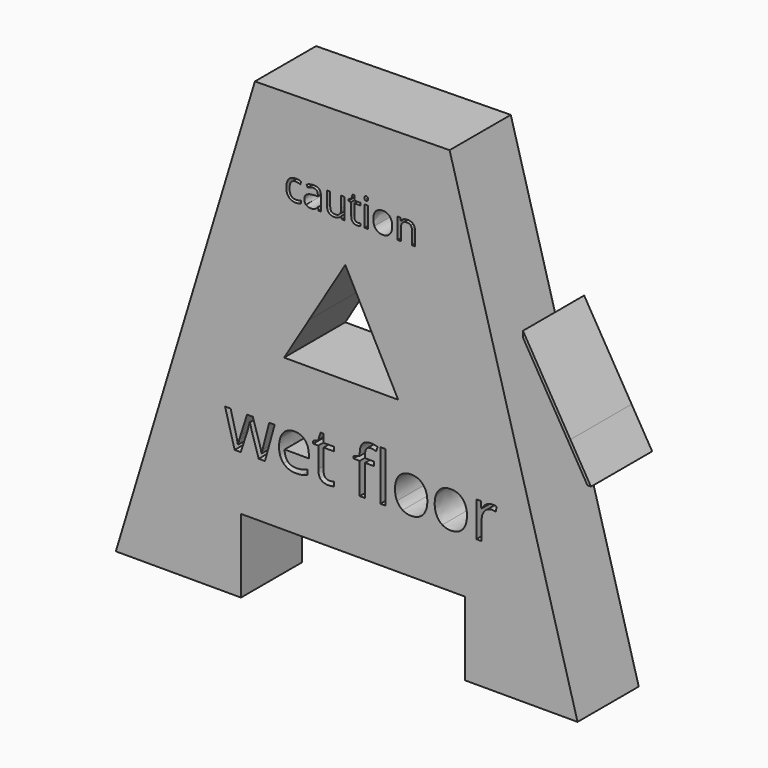
from build123d import *

# Parameters (mm, degrees)
F1_DEPTH = 12.7
F2_W     = 0.884249532
F2_H     = 8.2853670025
F2_W_2   = 0.5201468884
F2_H_2   = 3.4325685798
F3_DEPTH = 12.7


# Not quite as in the source:
# - a feature names something its author has since deleted; it is built from what else it names


with BuildPart() as f1:
    # F0 (on Front) → F1 (new body)
    with BuildSketch(Plane.XZ):
        with BuildLine():
            Line((9.6578345108, 21.5954678464), (6.4095085072, 27.0940973965))
            Line((6.4095085072, 27.0940973965), (6.4095085072, 26.0954775043))
            Line((6.4095085072, 26.0954775043), (9.3747755358, 21.0759982743))
            add(Edge.make_bspline(
                [(9.6578345108, 21.5954678464), (9.5118502558, 21.3402983679), (9.3747755358, 21.0759982743)],
                knots=[0.2874772556, 0.2874772556, 0.2874772556, 0.3442899073, 0.3442899073, 0.3442899073], degree=2))
        make_face()
        with BuildLine():
            Line((14.2873522737, 13.7588150149), (9.6578345108, 21.5954678464))
            add(Edge.make_bspline(
                [(9.6578345108, 21.5954678464), (9.5118502558, 21.3402983679), (9.3747755358, 21.0759982743)],
                knots=[0.2874772556, 0.2874772556, 0.2874772556, 0.3442899073, 0.3442899073, 0.3442899073], degree=2))
            Line((9.3747755358, 21.0759982743), (13.6974156478, 13.7588150149))
            Line((13.6974156478, 13.7588150149), (14.2873522737, 13.7588150149))
        make_face()
        Polygon((17.7024840034, 7.9778237518), (14.2873522737, 13.7588150149), (13.6974156478, 13.7588150149), (17.1125473775, 7.9778237518), align=None)
    extrude(amount=F1_DEPTH)


with BuildPart() as f3:
    # F2 (on Front) → F3 (new body)
    with BuildSketch(Plane.XZ):
        Polygon((-5.7727261446, 49.5300032198), (-38.1000004709, 49.0681789815), (-61.1909106374, -27.1318182349), (-40.4090918601, -27.1318182349), (-40.4090918601, -14.8936361074), (-3.2327286899, -14.8936361074), (-3.2327286899, -27.1318182349), (15.4709070921, -27.1318182349), align=None)
        Polygon((-47.3363660276, -7.9663638026), (-38.1000004709, 43.2954542339), (-7.398655434, 43.7340506074), (4.8490930349, -7.9663638026), align=None, mode=Mode.SUBTRACT)
        Polygon((-7.398655434, 43.7340506074), (-38.1000004709, 43.2954542339), (-47.3363660276, -7.9663638026), (4.8490930349, -7.9663638026), align=None)
        with BuildLine():
            Line((-36.4280137258, -5.8881817386), (-37.4775276213, -5.8881817386))
            Line((-37.4775276213, -5.8881817386), (-38.5474865926, -2.4653352841))
            add(Edge.make_bspline(
                [(-38.5474865926, -2.4653352841), (-38.649711972, -2.1501403642), (-38.9257204965, -1.0375874848)],
                knots=[0, 0, 0, 1, 1, 1], degree=2))
            Line((-38.9257204965, -1.0375874848), (-38.9683144046, -1.0375874848))
            add(Edge.make_bspline(
                [(-38.9683144046, -1.0375874848), (-39.1812839451, -1.9695421939), (-39.3414370395, -2.475557822)],
                knots=[0, 0, 0, 1, 1, 1], degree=2))
            Line((-39.3414370395, -2.475557822), (-40.443767381, -5.8881817386))
            Line((-40.443767381, -5.8881817386), (-41.4660211752, -5.8881817386))
            Line((-41.4660211752, -5.8881817386), (-43.0573295816, -0.0528163296))
            Line((-43.0573295816, -0.0528163296), (-42.1304861415, -0.0528163296))
            add(Edge.make_bspline(
                [(-42.1304861415, -0.0528163296), (-41.5665427983, -2.2523657436), (-41.2709410762, -3.4024012622)],
                knots=[0, 0, 0, 1, 1, 1], degree=2))
            add(Edge.make_bspline(
                [(-41.2709410762, -3.4024012622), (-40.975339354, -4.5524367807), (-40.9327454459, -4.9511157605)],
                knots=[0, 0, 0, 1, 1, 1], degree=2))
            Line((-40.9327454459, -4.9511157605), (-40.8901515378, -4.9511157605))
            add(Edge.make_bspline(
                [(-40.8901515378, -4.9511157605), (-40.8322238228, -4.6478471348), (-40.701886464, -4.1656840952)],
                knots=[0, 0, 0, 1, 1, 1], degree=2))
            add(Edge.make_bspline(
                [(-40.701886464, -4.1656840952), (-40.5715491053, -3.6835210556), (-40.4744349948, -3.4024012622)],
                knots=[0, 0, 0, 1, 1, 1], degree=2))
            Line((-40.4744349948, -3.4024012622), (-39.4044760235, -0.0528163296))
            Line((-39.4044760235, -0.0528163296), (-38.4469649695, -0.0528163296))
            Line((-38.4469649695, -0.0528163296), (-37.402562343, -3.4024012622))
            add(Edge.make_bspline(
                [(-37.402562343, -3.4024012622), (-37.1044049864, -4.317318408), (-36.9987720943, -4.9408932225)],
                knots=[0, 0, 0, 1, 1, 1], degree=2))
            Line((-36.9987720943, -4.9408932225), (-36.9561781862, -4.9408932225))
            add(Edge.make_bspline(
                [(-36.9561781862, -4.9408932225), (-36.934029354, -4.7483687579), (-36.8411746343, -4.3488379)],
                knots=[0, 0, 0, 1, 1, 1], degree=2))
            add(Edge.make_bspline(
                [(-36.8411746343, -4.3488379), (-36.7483199147, -3.9493070421), (-35.7311773894, -0.0528163296)],
                knots=[0, 0, 0, 1, 1, 1], degree=2))
            Line((-35.7311773894, -0.0528163296), (-34.8162602435, -0.0528163296))
            Line((-34.8162602435, -0.0528163296), (-36.4280137258, -5.8881817386))
        make_face(mode=Mode.SUBTRACT)
        with BuildLine():
            add(Edge.make_bspline(
                [(-30.2876759349, -5.9069230581), (-30.7050962343, -5.995518387), (-31.2962996786, -5.995518387)],
                knots=[0, 0, 0, 1, 1, 1], degree=2))
            add(Edge.make_bspline(
                [(-31.2962996786, -5.995518387), (-32.5894507284, -5.995518387), (-33.3382516327, -5.206679209)],
                knots=[0, 0, 0, 1, 1, 1], degree=2))
            add(Edge.make_bspline(
                [(-33.3382516327, -5.206679209), (-34.087052537, -4.4178400311), (-34.087052537, -3.0190560893)],
                knots=[0, 0, 0, 1, 1, 1], degree=2))
            add(Edge.make_bspline(
                [(-34.087052537, -3.0190560893), (-34.087052537, -1.6066420969), (-33.3919199569, -0.7760608891)],
                knots=[0, 0, 0, 1, 1, 1], degree=2))
            add(Edge.make_bspline(
                [(-33.3919199569, -0.7760608891), (-32.6967873768, 0.0545203188), (-31.524603026, 0.0545203188)],
                knots=[0, 0, 0, 1, 1, 1], degree=2))
            add(Edge.make_bspline(
                [(-31.524603026, 0.0545203188), (-30.4290877098, 0.0545203188), (-29.7901790884, -0.6670204843)],
                knots=[0, 0, 0, 1, 1, 1], degree=2))
            add(Edge.make_bspline(
                [(-29.7901790884, -0.6670204843), (-29.151270467, -1.3885612875), (-29.151270467, -2.5709681762)],
                knots=[0, 0, 0, 1, 1, 1], degree=2))
            Line((-29.151270467, -2.5709681762), (-29.151270467, -3.1298002504))
            Line((-29.151270467, -3.1298002504), (-33.1704316348, -3.1298002504))
            add(Edge.make_bspline(
                [(-33.1704316348, -3.1298002504), (-33.1431715336, -4.1571653136), (-32.650785956, -4.6895891648)],
                knots=[0, 0, 0, 1, 1, 1], degree=2))
            add(Edge.make_bspline(
                [(-32.650785956, -4.6895891648), (-32.1584003784, -5.222013016), (-31.2639283085, -5.222013016)],
                knots=[0, 0, 0, 1, 1, 1], degree=2))
            add(Edge.make_bspline(
                [(-31.2639283085, -5.222013016), (-30.3217510614, -5.222013016), (-29.4017226466, -4.8284453052)],
                knots=[0, 0, 0, 1, 1, 1], degree=2))
            Line((-29.4017226466, -4.8284453052), (-29.4017226466, -5.6172844831))
            add(Edge.make_bspline(
                [(-29.4017226466, -5.6172844831), (-29.8702556356, -5.8183277293), (-30.2876759349, -5.9069230581)],
                knots=[0, 0, 0, 1, 1, 1], degree=2))
        make_face(mode=Mode.SUBTRACT)
        with BuildLine():
            add(Edge.make_bspline(
                [(-26.4457054248, -4.9826352525), (-26.1952532452, -5.2646069241), (-25.7590916263, -5.2646069241)],
                knots=[0, 0, 0, 1, 1, 1], degree=2))
            add(Edge.make_bspline(
                [(-25.7590916263, -5.2646069241), (-25.5239732537, -5.2646069241), (-25.3058924442, -5.2305317976)],
                knots=[0, 0, 0, 1, 1, 1], degree=2))
            add(Edge.make_bspline(
                [(-25.3058924442, -5.2305317976), (-25.0878116348, -5.1964566711), (-24.9600299105, -5.158974032)],
                knots=[0, 0, 0, 1, 1, 1], degree=2))
            Line((-24.9600299105, -5.158974032), (-24.9600299105, -5.8353652925))
            add(Edge.make_bspline(
                [(-24.9600299105, -5.8353652925), (-25.1031454417, -5.9035155455), (-25.3825614788, -5.9495169662)],
                knots=[0, 0, 0, 1, 1, 1], degree=2))
            add(Edge.make_bspline(
                [(-25.3825614788, -5.9495169662), (-25.6619775159, -5.995518387), (-25.8868733506, -5.995518387)],
                knots=[0, 0, 0, 1, 1, 1], degree=2))
            add(Edge.make_bspline(
                [(-25.8868733506, -5.995518387), (-27.5787033801, -5.995518387), (-27.5787033801, -4.211685516)],
                knots=[0, 0, 0, 1, 1, 1], degree=2))
            Line((-27.5787033801, -4.211685516), (-27.5787033801, -0.7394301281))
            Line((-27.5787033801, -0.7394301281), (-28.4152477351, -0.7394301281))
            Line((-28.4152477351, -0.7394301281), (-28.4152477351, -0.3134910472))
            Line((-28.4152477351, -0.3134910472), (-27.5787033801, 0.0545203188))
            Line((-27.5787033801, 0.0545203188), (-27.2072845016, 1.2999661915))
            Line((-27.2072845016, 1.2999661915), (-26.6961576044, 1.2999661915))
            Line((-26.6961576044, 1.2999661915), (-26.6961576044, -0.0528163296))
            Line((-26.6961576044, -0.0528163296), (-25.0026238186, -0.0528163296))
            Line((-25.0026238186, -0.0528163296), (-25.0026238186, -0.7394301281))
            Line((-25.0026238186, -0.7394301281), (-26.6961576044, -0.7394301281))
            Line((-26.6961576044, -0.7394301281), (-26.6961576044, -4.1742028768))
            add(Edge.make_bspline(
                [(-26.6961576044, -4.1742028768), (-26.6961576044, -4.7006635809), (-26.4457054248, -4.9826352525)],
                knots=[0, 0, 0, 1, 1, 1], degree=2))
        make_face(mode=Mode.SUBTRACT)
        with BuildLine():
            Line((-18.3307140547, -0.0528163296), (-18.3307140547, -0.7394301281))
            Line((-18.3307140547, -0.7394301281), (-19.816389569, -0.7394301281))
            Line((-19.816389569, -0.7394301281), (-19.816389569, -5.8881817386))
            Line((-19.816389569, -5.8881817386), (-20.7006391011, -5.8881817386))
            Line((-20.7006391011, -5.8881817386), (-20.7006391011, -0.7394301281))
            Line((-20.7006391011, -0.7394301281), (-21.7433379712, -0.7394301281))
            Line((-21.7433379712, -0.7394301281), (-21.7433379712, -0.3407511483))
            Line((-21.7433379712, -0.3407511483), (-20.7006391011, -0.0204449595))
            Line((-20.7006391011, -0.0204449595), (-20.7006391011, 0.303268742))
            add(Edge.make_bspline(
                [(-20.7006391011, 0.303268742), (-20.7006391011, 2.455112979), (-18.8213958759, 2.455112979)],
                knots=[0, 0, 0, 1, 1, 1], degree=2))
            add(Edge.make_bspline(
                [(-18.8213958759, 2.455112979), (-18.3579741559, 2.455112979), (-17.7343993414, 2.2694035397)],
                knots=[0, 0, 0, 1, 1, 1], degree=2))
            Line((-17.7343993414, 2.2694035397), (-17.9644064451, 1.560640909))
            add(Edge.make_bspline(
                [(-17.9644064451, 1.560640909), (-18.4755333422, 1.7259052724), (-18.8367296828, 1.7259052724)],
                knots=[0, 0, 0, 1, 1, 1], degree=2))
            add(Edge.make_bspline(
                [(-18.8367296828, 1.7259052724), (-19.337634042, 1.7259052724), (-19.5770118055, 1.3928209111)],
                knots=[0, 0, 0, 1, 1, 1], degree=2))
            add(Edge.make_bspline(
                [(-19.5770118055, 1.3928209111), (-19.816389569, 1.0597365498), (-19.816389569, 0.3254175743)],
                knots=[0, 0, 0, 1, 1, 1], degree=2))
            Line((-19.816389569, 0.3254175743), (-19.816389569, -0.0528163296))
            Line((-19.816389569, -0.0528163296), (-18.3307140547, -0.0528163296))
        make_face(mode=Mode.SUBTRACT)
        with Locations((-16.8237415863, -1.7454982373)):
            Rectangle(F2_W, F2_H, mode=Mode.SUBTRACT)
        with BuildLine():
            add(Edge.make_bspline(
                [(-10.1927219742, -0.7607270822), (-9.471181171, -1.5759744831), (-9.471181171, -2.964535887)],
                knots=[0, 0, 0, 1, 1, 1], degree=2))
            add(Edge.make_bspline(
                [(-9.471181171, -2.964535887), (-9.471181171, -4.3922836863), (-10.1893144615, -5.1939010366)],
                knots=[0, 0, 0, 1, 1, 1], degree=2))
            add(Edge.make_bspline(
                [(-10.1893144615, -5.1939010366), (-10.907447752, -5.995518387), (-12.1750424569, -5.995518387)],
                knots=[0, 0, 0, 1, 1, 1], degree=2))
            add(Edge.make_bspline(
                [(-12.1750424569, -5.995518387), (-12.9587703658, -5.995518387), (-13.5653076171, -5.627507021)],
                knots=[0, 0, 0, 1, 1, 1], degree=2))
            add(Edge.make_bspline(
                [(-13.5653076171, -5.627507021), (-14.1718448683, -5.2594956551), (-14.5023735952, -4.5728818566)],
                knots=[0, 0, 0, 1, 1, 1], degree=2))
            add(Edge.make_bspline(
                [(-14.5023735952, -4.5728818566), (-14.832902322, -3.8862680581), (-14.832902322, -2.964535887)],
                knots=[0, 0, 0, 1, 1, 1], degree=2))
            add(Edge.make_bspline(
                [(-14.832902322, -2.964535887), (-14.832902322, -1.538491844), (-14.1190284223, -0.7419857626)],
                knots=[0, 0, 0, 1, 1, 1], degree=2))
            add(Edge.make_bspline(
                [(-14.1190284223, -0.7419857626), (-13.4051545226, 0.0545203188), (-12.1375598178, 0.0545203188)],
                knots=[0, 0, 0, 1, 1, 1], degree=2))
            add(Edge.make_bspline(
                [(-12.1375598178, 0.0545203188), (-10.9142627773, 0.0545203188), (-10.1927219742, -0.7607270822)],
                knots=[0, 0, 0, 1, 1, 1], degree=2))
        make_face(mode=Mode.SUBTRACT)
        with BuildLine():
            add(Edge.make_bspline(
                [(-3.6060000264, -0.7607270822), (-2.8844592233, -1.5759744831), (-2.8844592233, -2.964535887)],
                knots=[0, 0, 0, 1, 1, 1], degree=2))
            add(Edge.make_bspline(
                [(-2.8844592233, -2.964535887), (-2.8844592233, -4.3922836863), (-3.6025925138, -5.1939010366)],
                knots=[0, 0, 0, 1, 1, 1], degree=2))
            add(Edge.make_bspline(
                [(-3.6025925138, -5.1939010366), (-4.3207258043, -5.995518387), (-5.5883205092, -5.995518387)],
                knots=[0, 0, 0, 1, 1, 1], degree=2))
            add(Edge.make_bspline(
                [(-5.5883205092, -5.995518387), (-6.3720484181, -5.995518387), (-6.9785856694, -5.627507021)],
                knots=[0, 0, 0, 1, 1, 1], degree=2))
            add(Edge.make_bspline(
                [(-6.9785856694, -5.627507021), (-7.5851229206, -5.2594956551), (-7.9156516474, -4.5728818566)],
                knots=[0, 0, 0, 1, 1, 1], degree=2))
            add(Edge.make_bspline(
                [(-7.9156516474, -4.5728818566), (-8.2461803742, -3.8862680581), (-8.2461803742, -2.964535887)],
                knots=[0, 0, 0, 1, 1, 1], degree=2))
            add(Edge.make_bspline(
                [(-8.2461803742, -2.964535887), (-8.2461803742, -1.538491844), (-7.5323064746, -0.7419857626)],
                knots=[0, 0, 0, 1, 1, 1], degree=2))
            add(Edge.make_bspline(
                [(-7.5323064746, -0.7419857626), (-6.8184325749, 0.0545203188), (-5.55083787, 0.0545203188)],
                knots=[0, 0, 0, 1, 1, 1], degree=2))
            add(Edge.make_bspline(
                [(-5.55083787, 0.0545203188), (-4.3275408296, 0.0545203188), (-3.6060000264, -0.7607270822)],
                knots=[0, 0, 0, 1, 1, 1], degree=2))
        make_face(mode=Mode.SUBTRACT)
        with BuildLine():
            add(Edge.make_bspline(
                [(0.322010178, -0.254711454), (0.7803206291, 0.0545203188), (1.3289301654, 0.0545203188)],
                knots=[0, 0, 0, 1, 1, 1], degree=2))
            add(Edge.make_bspline(
                [(1.3289301654, 0.0545203188), (1.7173866072, 0.0545203188), (2.0257665018, -0.0102224215)],
                knots=[0, 0, 0, 1, 1, 1], degree=2))
            Line((2.0257665018, -0.0102224215), (1.9030960465, -0.8297292133))
            add(Edge.make_bspline(
                [(1.9030960465, -0.8297292133), (1.5418997058, -0.749652666), (1.2641874251, -0.749652666)],
                knots=[0, 0, 0, 1, 1, 1], degree=2))
            add(Edge.make_bspline(
                [(1.2641874251, -0.749652666), (0.5554247944, -0.749652666), (0.0528166789, -1.3246704253)],
                knots=[0, 0, 0, 1, 1, 1], degree=2))
            add(Edge.make_bspline(
                [(0.0528166789, -1.3246704253), (-0.4497914366, -1.8996881846), (-0.4497914366, -2.7566776155)],
                knots=[0, 0, 0, 1, 1, 1], degree=2))
            Line((-0.4497914366, -2.7566776155), (-0.4497914366, -5.8881817386))
            Line((-0.4497914366, -5.8881817386), (-1.3340409687, -5.8881817386))
            Line((-1.3340409687, -5.8881817386), (-1.3340409687, -0.0528163296))
            Line((-1.3340409687, -0.0528163296), (-0.6048332621, -0.0528163296))
            Line((-0.6048332621, -0.0528163296), (-0.5026078827, -1.1329978389))
            Line((-0.5026078827, -1.1329978389), (-0.4600139746, -1.1329978389))
            add(Edge.make_bspline(
                [(-0.4600139746, -1.1329978389), (-0.1363002731, -0.5639432268), (0.322010178, -0.254711454)],
                knots=[0, 0, 0, 1, 1, 1], degree=2))
        make_face(mode=Mode.SUBTRACT)
        Polygon((-29.1155879012, 17.1363315055), (-23.0909101665, 27.1318182349), (-14.3163632601, 10.2754551917), (-20.3199982643, 10.2754551917), (-28.6327283829, 10.2754551917), (-33.2509111613, 10.2754551917), align=None, mode=Mode.SUBTRACT)
        with BuildLine():
            add(Edge.make_bspline(
                [(-30.460759066, 33.7135282268), (-30.8045170289, 33.5341326718), (-31.3276705468, 33.5341326718)],
                knots=[0, 0, 0, 1, 1, 1], degree=2))
            add(Edge.make_bspline(
                [(-31.3276705468, 33.5341326718), (-32.0733146412, 33.5341326718), (-32.4822162414, 33.9931447622)],
                knots=[0, 0, 0, 1, 1, 1], degree=2))
            add(Edge.make_bspline(
                [(-32.4822162414, 33.9931447622), (-32.8911178415, 34.4521568525), (-32.8911178415, 35.2920086686)],
                knots=[0, 0, 0, 1, 1, 1], degree=2))
            add(Edge.make_bspline(
                [(-32.8911178415, 35.2920086686), (-32.8911178415, 36.1529068905), (-32.4757018777, 36.6229432887)],
                knots=[0, 0, 0, 1, 1, 1], degree=2))
            add(Edge.make_bspline(
                [(-32.4757018777, 36.6229432887), (-32.0602859138, 37.092979687), (-31.2935954134, 37.092979687)],
                knots=[0, 0, 0, 1, 1, 1], degree=2))
            add(Edge.make_bspline(
                [(-31.2935954134, 37.092979687), (-31.0460495918, 37.092979687), (-30.7985037701, 37.0393614624)],
                knots=[0, 0, 0, 1, 1, 1], degree=2))
            add(Edge.make_bspline(
                [(-30.7985037701, 37.0393614624), (-30.5509579484, 36.9857432379), (-30.4106485758, 36.913584132)],
                knots=[0, 0, 0, 1, 1, 1], degree=2))
            Line((-30.4106485758, 36.913584132), (-30.5699999347, 36.4726118181))
            add(Edge.make_bspline(
                [(-30.5699999347, 36.4726118181), (-30.7423800211, 36.5417642946), (-30.9458286113, 36.5868637358)],
                knots=[0, 0, 0, 1, 1, 1], degree=2))
            add(Edge.make_bspline(
                [(-30.9458286113, 36.5868637358), (-31.1492772016, 36.631963177), (-31.3056219311, 36.631963177)],
                knots=[0, 0, 0, 1, 1, 1], degree=2))
            add(Edge.make_bspline(
                [(-31.3056219311, 36.631963177), (-32.3519289668, 36.631963177), (-32.3519289668, 35.2980219274)],
                knots=[0, 0, 0, 1, 1, 1], degree=2))
            add(Edge.make_bspline(
                [(-32.3519289668, 35.2980219274), (-32.3519289668, 34.6656275409), (-32.0968665716, 34.3273817319)],
                knots=[0, 0, 0, 1, 1, 1], degree=2))
            add(Edge.make_bspline(
                [(-32.0968665716, 34.3273817319), (-31.8418041764, 33.9891359229), (-31.3406992742, 33.9891359229)],
                knots=[0, 0, 0, 1, 1, 1], degree=2))
            add(Edge.make_bspline(
                [(-31.3406992742, 33.9891359229), (-30.911753478, 33.9891359229), (-30.460759066, 34.1735425269)],
                knots=[0, 0, 0, 1, 1, 1], degree=2))
            Line((-30.460759066, 34.1735425269), (-30.460759066, 33.7135282268))
        make_face(mode=Mode.SUBTRACT)
        with BuildLine():
            Line((-27.1494578725, 33.5972718894), (-27.5353086472, 33.5972718894))
            Line((-27.5353086472, 33.5972718894), (-27.638536257, 34.086350274))
            Line((-27.638536257, 34.086350274), (-27.6635915022, 34.086350274))
            add(Edge.make_bspline(
                [(-27.6635915022, 34.086350274), (-27.9201572121, 33.763638717), (-28.1752196073, 33.6488856944)],
                knots=[0, 0, 0, 1, 1, 1], degree=2))
            add(Edge.make_bspline(
                [(-28.1752196073, 33.6488856944), (-28.4302820025, 33.5341326718), (-28.8131261477, 33.5341326718)],
                knots=[0, 0, 0, 1, 1, 1], degree=2))
            add(Edge.make_bspline(
                [(-28.8131261477, 33.5341326718), (-29.3232509381, 33.5341326718), (-29.6128895716, 33.7977138503)],
                knots=[0, 0, 0, 1, 1, 1], degree=2))
            add(Edge.make_bspline(
                [(-29.6128895716, 33.7977138503), (-29.902528205, 34.0612950289), (-29.902528205, 34.5463645741)],
                knots=[0, 0, 0, 1, 1, 1], degree=2))
            add(Edge.make_bspline(
                [(-29.902528205, 34.5463645741), (-29.902528205, 35.5856561412), (-28.2398621396, 35.6357666315)],
                knots=[0, 0, 0, 1, 1, 1], degree=2))
            Line((-28.2398621396, 35.6357666315), (-27.6575782433, 35.6548086177))
            Line((-27.6575782433, 35.6548086177), (-27.6575782433, 35.8682793061))
            add(Edge.make_bspline(
                [(-27.6575782433, 35.8682793061), (-27.6575782433, 36.2721698572), (-27.8309605395, 36.4645941396)],
                knots=[0, 0, 0, 1, 1, 1], degree=2))
            add(Edge.make_bspline(
                [(-27.8309605395, 36.4645941396), (-28.0043428356, 36.6570184221), (-28.3871869809, 36.6570184221)],
                knots=[0, 0, 0, 1, 1, 1], degree=2))
            add(Edge.make_bspline(
                [(-28.3871869809, 36.6570184221), (-28.8161327771, 36.6570184221), (-29.3573260715, 36.3944394533)],
                knots=[0, 0, 0, 1, 1, 1], degree=2))
            Line((-29.3573260715, 36.3944394533), (-29.5176796402, 36.7923167457))
            add(Edge.make_bspline(
                [(-29.5176796402, 36.7923167457), (-29.2641205597, 36.9296194888), (-28.9619543037, 37.0077918536)],
                knots=[0, 0, 0, 1, 1, 1], degree=2))
            add(Edge.make_bspline(
                [(-28.9619543037, 37.0077918536), (-28.6597880477, 37.0859642183), (-28.3551162671, 37.0859642183)],
                knots=[0, 0, 0, 1, 1, 1], degree=2))
            add(Edge.make_bspline(
                [(-28.3551162671, 37.0859642183), (-27.7417638669, 37.0859642183), (-27.4456108697, 36.8138642564)],
                knots=[0, 0, 0, 1, 1, 1], degree=2))
            add(Edge.make_bspline(
                [(-27.4456108697, 36.8138642564), (-27.1494578725, 36.5417642946), (-27.1494578725, 35.940438412)],
                knots=[0, 0, 0, 1, 1, 1], degree=2))
            Line((-27.1494578725, 35.940438412), (-27.1494578725, 33.5972718894))
        make_face(mode=Mode.SUBTRACT)
        with BuildLine():
            Line((-26.1161795643, 37.0298404693), (-25.590019417, 37.0298404693))
            Line((-25.590019417, 37.0298404693), (-25.590019417, 34.8029302841))
            add(Edge.make_bspline(
                [(-25.590019417, 34.8029302841), (-25.590019417, 34.383004376), (-25.3990984493, 34.1765491564)],
                knots=[0, 0, 0, 1, 1, 1], degree=2))
            add(Edge.make_bspline(
                [(-25.3990984493, 34.1765491564), (-25.2081774815, 33.9700939367), (-24.801280301, 33.9700939367)],
                knots=[0, 0, 0, 1, 1, 1], degree=2))
            add(Edge.make_bspline(
                [(-24.801280301, 33.9700939367), (-24.2620914263, 33.9700939367), (-24.0135433948, 34.2642425142)],
                knots=[0, 0, 0, 1, 1, 1], degree=2))
            add(Edge.make_bspline(
                [(-24.0135433948, 34.2642425142), (-23.7649953633, 34.5583910918), (-23.7649953633, 35.2258628215)],
                knots=[0, 0, 0, 1, 1, 1], degree=2))
            Line((-23.7649953633, 35.2258628215), (-23.7649953633, 37.0298404693))
            Line((-23.7649953633, 37.0298404693), (-23.2448484749, 37.0298404693))
            Line((-23.2448484749, 37.0298404693), (-23.2448484749, 33.5972718894))
            Line((-23.2448484749, 33.5972718894), (-23.6737942711, 33.5972718894))
            Line((-23.6737942711, 33.5972718894), (-23.7489600064, 34.0572861896))
            Line((-23.7489600064, 34.0572861896), (-23.777021881, 34.0572861896))
            add(Edge.make_bspline(
                [(-23.777021881, 34.0572861896), (-23.9363732398, 33.8037271091), (-24.2199986145, 33.6689298905)],
                knots=[0, 0, 0, 1, 1, 1], degree=2))
            add(Edge.make_bspline(
                [(-24.2199986145, 33.6689298905), (-24.5036239891, 33.5341326718), (-24.8674261481, 33.5341326718)],
                knots=[0, 0, 0, 1, 1, 1], degree=2))
            add(Edge.make_bspline(
                [(-24.8674261481, 33.5341326718), (-25.4938072758, 33.5341326718), (-25.80499342, 33.8317889837)],
                knots=[0, 0, 0, 1, 1, 1], degree=2))
            add(Edge.make_bspline(
                [(-25.80499342, 33.8317889837), (-26.1161795643, 34.1294452955), (-26.1161795643, 34.7838882978)],
                knots=[0, 0, 0, 1, 1, 1], degree=2))
            Line((-26.1161795643, 34.7838882978), (-26.1161795643, 37.0298404693))
        make_face(mode=Mode.SUBTRACT)
        with BuildLine():
            add(Edge.make_bspline(
                [(-21.4378641977, 34.1299464005), (-21.2905393564, 33.9640806778), (-21.0339736465, 33.9640806778)],
                knots=[0, 0, 0, 1, 1, 1], degree=2))
            add(Edge.make_bspline(
                [(-21.0339736465, 33.9640806778), (-20.8956686935, 33.9640806778), (-20.7673858386, 33.9841248739)],
                knots=[0, 0, 0, 1, 1, 1], degree=2))
            add(Edge.make_bspline(
                [(-20.7673858386, 33.9841248739), (-20.6391029836, 34.00416907), (-20.5639372483, 34.0262176857)],
                knots=[0, 0, 0, 1, 1, 1], degree=2))
            Line((-20.5639372483, 34.0262176857), (-20.5639372483, 33.6283403934))
            add(Edge.make_bspline(
                [(-20.5639372483, 33.6283403934), (-20.6481228718, 33.5882520012), (-20.8124852797, 33.5611923365)],
                knots=[0, 0, 0, 1, 1, 1], degree=2))
            add(Edge.make_bspline(
                [(-20.8124852797, 33.5611923365), (-20.9768476877, 33.5341326718), (-21.1091393818, 33.5341326718)],
                knots=[0, 0, 0, 1, 1, 1], degree=2))
            add(Edge.make_bspline(
                [(-21.1091393818, 33.5341326718), (-22.1043337175, 33.5341326718), (-22.1043337175, 34.5834463369)],
                knots=[0, 0, 0, 1, 1, 1], degree=2))
            Line((-22.1043337175, 34.5834463369), (-22.1043337175, 36.6259499181))
            Line((-22.1043337175, 36.6259499181), (-22.5964187315, 36.6259499181))
            Line((-22.5964187315, 36.6259499181), (-22.5964187315, 36.8765023692))
            Line((-22.5964187315, 36.8765023692), (-22.1043337175, 37.092979687))
            Line((-22.1043337175, 37.092979687), (-21.8858519802, 37.8255950539))
            Line((-21.8858519802, 37.8255950539), (-21.5851890389, 37.8255950539))
            Line((-21.5851890389, 37.8255950539), (-21.5851890389, 37.0298404693))
            Line((-21.5851890389, 37.0298404693), (-20.5889924934, 37.0298404693))
            Line((-20.5889924934, 37.0298404693), (-20.5889924934, 36.6259499181))
            Line((-20.5889924934, 36.6259499181), (-21.5851890389, 36.6259499181))
            Line((-21.5851890389, 36.6259499181), (-21.5851890389, 34.6054949526))
            add(Edge.make_bspline(
                [(-21.5851890389, 34.6054949526), (-21.5851890389, 34.2958121231), (-21.4378641977, 34.1299464005)],
                knots=[0, 0, 0, 1, 1, 1], degree=2))
        make_face(mode=Mode.SUBTRACT)
        with Locations((-19.6183522979, 35.3135561794)):
            Rectangle(F2_W_2, F2_H_2, mode=Mode.SUBTRACT)
        with BuildLine():
            add(Edge.make_bspline(
                [(-19.8348296156, 37.6983144088), (-19.9225229735, 37.7845044519), (-19.9225229735, 37.9598911677)],
                knots=[0, 0, 0, 1, 1, 1], degree=2))
            add(Edge.make_bspline(
                [(-19.9225229735, 37.9598911677), (-19.9225229735, 38.1382845129), (-19.8348296156, 38.2214679266)],
                knots=[0, 0, 0, 1, 1, 1], degree=2))
            add(Edge.make_bspline(
                [(-19.8348296156, 38.2214679266), (-19.7471362577, 38.3046513404), (-19.6148445636, 38.3046513404)],
                knots=[0, 0, 0, 1, 1, 1], degree=2))
            add(Edge.make_bspline(
                [(-19.6148445636, 38.3046513404), (-19.489568338, 38.3046513404), (-19.3988683507, 38.2199646119)],
                knots=[0, 0, 0, 1, 1, 1], degree=2))
            add(Edge.make_bspline(
                [(-19.3988683507, 38.2199646119), (-19.3081683634, 38.1352778835), (-19.3081683634, 37.9598911677)],
                knots=[0, 0, 0, 1, 1, 1], degree=2))
            add(Edge.make_bspline(
                [(-19.3081683634, 37.9598911677), (-19.3081683634, 37.7845044519), (-19.3988683507, 37.6983144088)],
                knots=[0, 0, 0, 1, 1, 1], degree=2))
            add(Edge.make_bspline(
                [(-19.3988683507, 37.6983144088), (-19.489568338, 37.6121243656), (-19.6148445636, 37.6121243656)],
                knots=[0, 0, 0, 1, 1, 1], degree=2))
            add(Edge.make_bspline(
                [(-19.6148445636, 37.6121243656), (-19.7471362577, 37.6121243656), (-19.8348296156, 37.6983144088)],
                knots=[0, 0, 0, 1, 1, 1], degree=2))
        make_face(mode=Mode.SUBTRACT)
        with BuildLine():
            add(Edge.make_bspline(
                [(-15.7177517394, 36.6134222956), (-15.2933158873, 36.1338649042), (-15.2933158873, 35.3170639137)],
                knots=[0, 0, 0, 1, 1, 1], degree=2))
            add(Edge.make_bspline(
                [(-15.2933158873, 35.3170639137), (-15.2933158873, 34.4772120977), (-15.7157473198, 34.0056723847)],
                knots=[0, 0, 0, 1, 1, 1], degree=2))
            add(Edge.make_bspline(
                [(-15.7157473198, 34.0056723847), (-16.1381787523, 33.5341326718), (-16.8838228468, 33.5341326718)],
                knots=[0, 0, 0, 1, 1, 1], degree=2))
            add(Edge.make_bspline(
                [(-16.8838228468, 33.5341326718), (-17.3448393568, 33.5341326718), (-17.7016260471, 33.7506099895)],
                knots=[0, 0, 0, 1, 1, 1], degree=2))
            add(Edge.make_bspline(
                [(-17.7016260471, 33.7506099895), (-18.0584127374, 33.9670873072), (-18.2528414395, 34.3709778584)],
                knots=[0, 0, 0, 1, 1, 1], degree=2))
            add(Edge.make_bspline(
                [(-18.2528414395, 34.3709778584), (-18.4472701415, 34.7748684095), (-18.4472701415, 35.3170639137)],
                knots=[0, 0, 0, 1, 1, 1], degree=2))
            add(Edge.make_bspline(
                [(-18.4472701415, 35.3170639137), (-18.4472701415, 36.1559135199), (-18.0273442335, 36.6244466034)],
                knots=[0, 0, 0, 1, 1, 1], degree=2))
            add(Edge.make_bspline(
                [(-18.0273442335, 36.6244466034), (-17.6074183255, 37.092979687), (-16.8617742311, 37.092979687)],
                knots=[0, 0, 0, 1, 1, 1], degree=2))
            add(Edge.make_bspline(
                [(-16.8617742311, 37.092979687), (-16.1421875916, 37.092979687), (-15.7177517394, 36.6134222956)],
                knots=[0, 0, 0, 1, 1, 1], degree=2))
        make_face(mode=Mode.SUBTRACT)
        with BuildLine():
            Line((-11.5119782956, 33.5972718894), (-12.032125184, 33.5972718894))
            Line((-12.032125184, 33.5972718894), (-12.032125184, 35.8181688158))
            add(Edge.make_bspline(
                [(-12.032125184, 35.8181688158), (-12.032125184, 36.2370925141), (-12.2230461517, 36.4440488387)],
                knots=[0, 0, 0, 1, 1, 1], degree=2))
            add(Edge.make_bspline(
                [(-12.2230461517, 36.4440488387), (-12.4139671195, 36.6510051632), (-12.8218665098, 36.6510051632)],
                knots=[0, 0, 0, 1, 1, 1], degree=2))
            add(Edge.make_bspline(
                [(-12.8218665098, 36.6510051632), (-13.3600531747, 36.6510051632), (-13.6106056258, 36.3598632151)],
                knots=[0, 0, 0, 1, 1, 1], degree=2))
            add(Edge.make_bspline(
                [(-13.6106056258, 36.3598632151), (-13.8611580769, 36.0687212669), (-13.8611580769, 35.3982429078)],
                knots=[0, 0, 0, 1, 1, 1], degree=2))
            Line((-13.8611580769, 35.3982429078), (-13.8611580769, 33.5972718894))
            Line((-13.8611580769, 33.5972718894), (-14.3813049654, 33.5972718894))
            Line((-14.3813049654, 33.5972718894), (-14.3813049654, 37.0298404693))
            Line((-14.3813049654, 37.0298404693), (-13.9583724279, 37.0298404693))
            Line((-13.9583724279, 37.0298404693), (-13.8741868044, 36.5598040711))
            Line((-13.8741868044, 36.5598040711), (-13.8491315593, 36.5598040711))
            add(Edge.make_bspline(
                [(-13.8491315593, 36.5598040711), (-13.6887779906, 36.8133631515), (-13.4006426718, 36.9531714193)],
                knots=[0, 0, 0, 1, 1, 1], degree=2))
            add(Edge.make_bspline(
                [(-13.4006426718, 36.9531714193), (-13.1125073531, 37.092979687), (-12.7587272921, 37.092979687)],
                knots=[0, 0, 0, 1, 1, 1], degree=2))
            add(Edge.make_bspline(
                [(-12.7587272921, 37.092979687), (-12.1383594233, 37.092979687), (-11.8251688594, 36.7938200604)],
                knots=[0, 0, 0, 1, 1, 1], degree=2))
            add(Edge.make_bspline(
                [(-11.8251688594, 36.7938200604), (-11.5119782956, 36.4946604338), (-11.5119782956, 35.8362085923)],
                knots=[0, 0, 0, 1, 1, 1], degree=2))
            Line((-11.5119782956, 35.8362085923), (-11.5119782956, 33.5972718894))
        make_face(mode=Mode.SUBTRACT)
    extrude(amount=F3_DEPTH)


solid = Compound([f1.part, f3.part])
